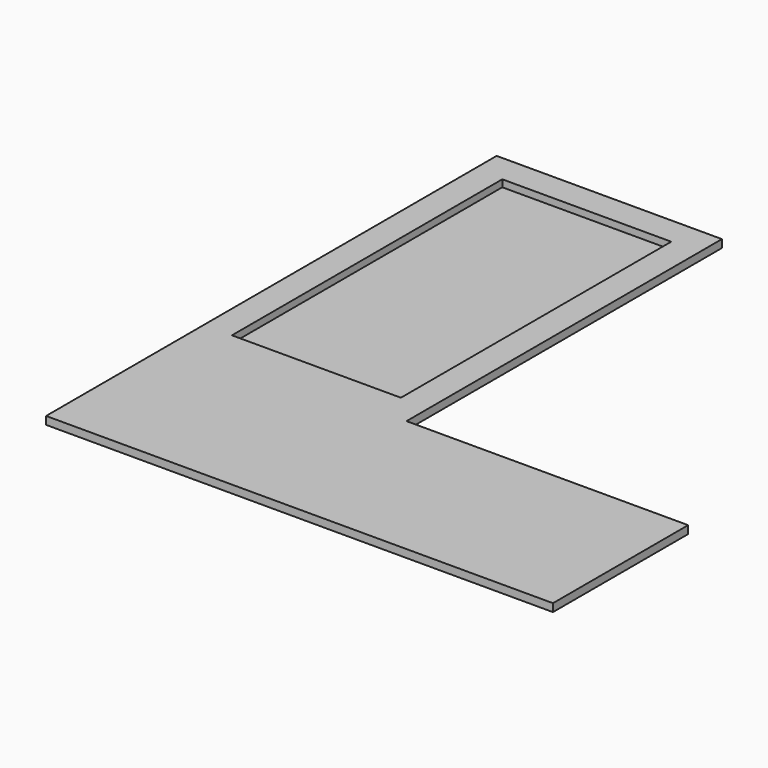
from build123d import *

# Parameters (mm, degrees)
F1_DEPTH = 28
F2_W     = 600
F2_H     = 1200
F3_DEPTH = 25


# Not quite as in the source:
# - the program builds the solid bodies; features that only make, move or delete a surface that nothing else refers to are left out


with BuildPart() as f1:
    # F0 (on Top) → F1 (new body)
    with BuildSketch(Plane.XY):
        Polygon((0, 2000), (0, 0), (1800, 0), (1800, 600), (800, 600), (800, 2000), align=None)
    extrude(amount=F1_DEPTH)

    # F2 (on face) → F3 (cut)
    with BuildSketch(Plane.XY.offset(28)):
        with Locations((400, 1300)):
            Rectangle(F2_W, F2_H)
    extrude(amount=-F3_DEPTH, mode=Mode.SUBTRACT)


solid = f1.part
